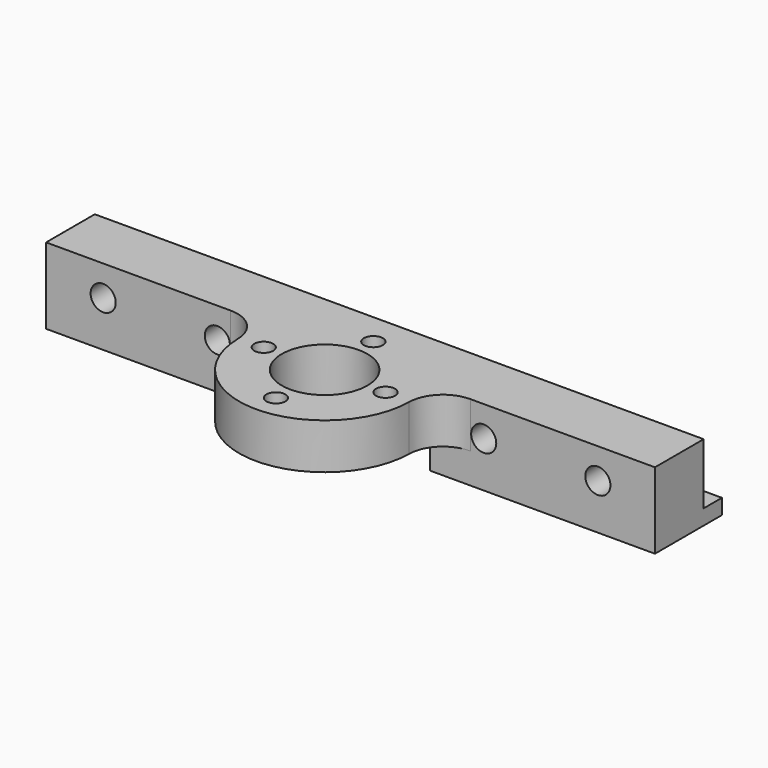
from build123d import *

# Parameters (mm, degrees)
F4_D      = 2.5
F3_R      = 5.625
F5_DEPTH  = 18.001
F7_DEPTH  = 10
F8_R      = 4.5
F9_W      = 80
F9_H      = 2
F10_DEPTH = 3
F12_D     = 3.3


with BuildPart() as f1:
    # F0 (on Front) → F1 (revolve)
    with BuildSketch(Plane.XZ):
        Polygon((5.125, 1.85), (3.5, 1.85), (3.5, -16.15), (5.125, -16.15), (5.125, -6), (11.25, -6), (11.25, 0), (5.125, 0), align=None)
    revolve(axis=Axis((0, 0, -12.1311874992), (0, 0, -1)))

    # F4 (through all)
    with Locations(Plane.XY):
        with Locations((0, 8), (8, 0), (0, -8), (-8, 0)):
            Hole(F4_D / 2)

    # F3 (on face) → F5 (cut, through all)
    with BuildSketch(Plane.XY.offset(1.85)):
        Circle(F3_R)
    extrude(amount=-F5_DEPTH, mode=Mode.SUBTRACT)

    # F6 (on face) → F7 (join)
    with BuildSketch(Plane.XY):
        with BuildLine():
            ThreePointArc((-10.416333328, 4.25), (0, 11.25), (10.416333328, 4.25))
            Line((10.416333328, 4.25), (40, 4.25))
            Line((40, 4.25), (40, 12.25))
            Line((40, 12.25), (-40, 12.25))
            Line((-40, 12.25), (-40, 4.25))
            Line((-40, 4.25), (-10.416333328, 4.25))
        make_face()
    extrude(amount=-F7_DEPTH)

    # F8
    f8_edges = [f1.edges().sort_by_distance(p)[0] for p in [
        (10.416333, 4.25, -3),
        (-10.416333, 4.25, -3),
    ]]
    fillet(f8_edges, radius=F8_R)

    # F9 (on face) → F10 (join)
    with BuildSketch(Plane(origin=(0, 12.25, 0), x_dir=(-1, 0, 0), z_dir=(0, 1, 0))):
        with Locations((0, -9)):
            Rectangle(F9_W, F9_H)
    extrude(amount=F10_DEPTH)

    # F12 (through all)
    with Locations(Plane(origin=(0, 12.25, 0), x_dir=(-1, 0, 0), z_dir=(0, 1, 0))):
        with Locations((-32.5, -4), (-17.5, -4), (17.5, -4), (32.5, -4)):
            Hole(F12_D / 2)


solid = f1.part
